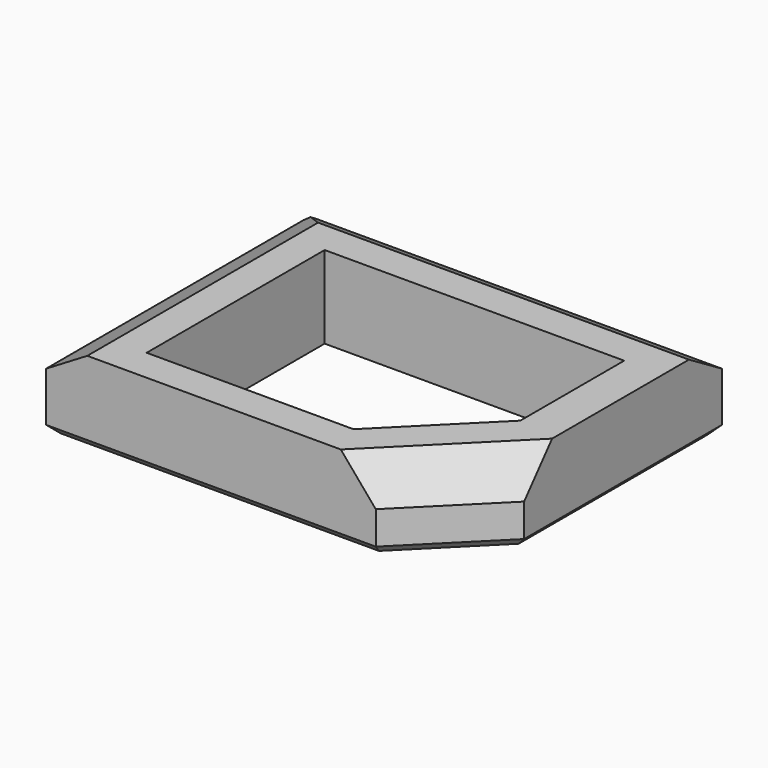
from build123d import *

# Parameters (mm, degrees)
F1_DEPTH    = 10
F2_C1_SIZE2 = 5
F2_C1_SIZE  = 3
F2_C2_SIZE2 = 5
F2_C2_SIZE  = 3
F2_C3_SIZE2 = 5
F2_C3_SIZE  = 3
F3_T1_DEPTH = 12.1433659759
F5_SIZE     = 1
F7_DEPTH    = 10.001


# Not quite as in the source:
# - a fillet or chamfer that OpenCascade refuses, or shapes differently, is made with other operations: its cross-section is extruded or revolved along the edge and cut away or added
# - two fillets or chamfers of one size are made in one step


with BuildPart() as f1:
    # F0 (on Top) → F1 (new body)
    with BuildSketch(Plane.XY):
        Polygon((50, 40), (0, 40), (0, 0), (40, 0), (50, 10), align=None)
    extrude(amount=F1_DEPTH)

    # F2: chamfer of 5 x 3 on 3 edges, made by hand

    # F2_c1
    f2_c1_edges = [f1.edges().sort_by_distance(p)[0] for p in [
        (25, 40, 10),
    ]]
    f2_c1_side = f1.faces().sort_by_distance((25, 40, 9.94))[0]
    chamfer(f2_c1_edges, length=F2_C1_SIZE, length2=F2_C1_SIZE2, reference=f2_c1_side)

    # F2_c2
    f2_c2_edges = [f1.edges().sort_by_distance(p)[0] for p in [
        (0, 17.5, 10),
    ]]
    f2_c2_side = f1.faces().sort_by_distance((0, 17.5, 9.94))[0]
    chamfer(f2_c2_edges, length=F2_C2_SIZE, length2=F2_C2_SIZE2, reference=f2_c2_side)

    # F2_c3
    f2_c3_edges = [f1.edges().sort_by_distance(p)[0] for p in [
        (45, 5, 10),
    ]]
    f2_c3_side = f1.faces().sort_by_distance((44.9575735931, 5.0424264069, 10))[0]
    chamfer(f2_c3_edges, length=F2_C3_SIZE, length2=F2_C3_SIZE2, reference=f2_c3_side)

    # F3: chamfer of 1 on 1 edges, made by hand

    # F3_s2 → F3_t1 (cut)
    with BuildSketch(Plane.XY.offset(-2.571682988)):
        Polygon((1, 40), (0, 39), (0, 40), align=None)
    extrude(amount=F3_T1_DEPTH, mode=Mode.SUBTRACT)

    # F5
    f5_edges = [f1.edges().sort_by_distance(p)[0] for p in [
        (50, 25, 0),
        (45, 5, 0),
        (20, 0, 0),
        (0, 19.5, 0),
        (0.5, 39.5, 0),
        (25.5, 40, 0),
    ]]
    chamfer(f5_edges, length=F5_SIZE)

    # F6 (on face) → F7 (cut, through all)
    with BuildSketch(Plane.XY.offset(10)):
        Polygon((9, 31), (9, 4), (34.1005050634, 4), (45.3436888701, 15.2431838067), (45.3436888701, 31), align=None)
    extrude(amount=-F7_DEPTH, mode=Mode.SUBTRACT)


solid = f1.part
